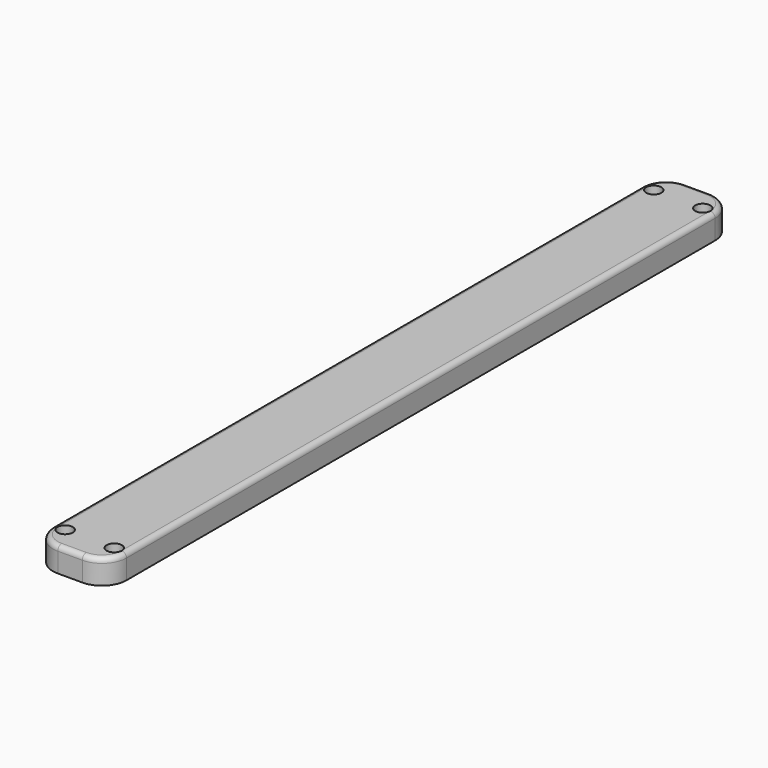
from build123d import *

# Parameters (mm, degrees)
F0_W         = 15
F0_H         = 160
F0_R         = 1.55
F1_DEPTH     = 5
F2_R         = 5
F3_T1_DEPTH  = 150
F3_T3_DEPTH  = 5
F3_T6_ANGLE  = 90
F3_T8_ANGLE  = 90
F3_T10_ANGLE = 90
F3_T12_ANGLE = 90


# Not quite as in the source:
# - a fillet or chamfer that OpenCascade refuses, or shapes differently, is made with other operations: its cross-section is extruded or revolved along the edge and cut away or added


with BuildPart() as f1:
    # F0 (on Top) → F1 (new body)
    with BuildSketch(Plane.XY):
        Rectangle(F0_W, F0_H)
        with Locations((-5, -75)):
            Circle(F0_R, mode=Mode.SUBTRACT)
        with BuildLine():
            ThreePointArc((6.55, -75), (5, -76.55), (3.45, -75))
            ThreePointArc((3.45, -75), (5, -73.45), (6.55, -75))
        make_face(mode=Mode.SUBTRACT)
        with Locations((-5, 75)):
            Circle(F0_R, mode=Mode.SUBTRACT)
        with BuildLine():
            ThreePointArc((6.55, 75), (5, 73.45), (3.45, 75))
            ThreePointArc((3.45, 75), (5, 76.55), (6.55, 75))
        make_face(mode=Mode.SUBTRACT)
    extrude(amount=F1_DEPTH)

    # F2
    f2_edges = [f1.edges().sort_by_distance(p)[0] for p in [
        (7.5, -80, 2.5),
        (-7.5, -80, 2.5),
        (7.5, 80, 2.5),
        (-7.5, 80, 2.5),
    ]]
    fillet(f2_edges, radius=F2_R)

    # F3: fillet of radius 1 on 8 edges, made by hand

    # F3_s2 → F3_t1 (cut)
    with BuildSketch(Plane.XZ.offset(-75)):
        with BuildLine():
            ThreePointArc((6.5, 5), (7.2071067812, 4.7071067812), (7.5, 4))
            Line((7.5, 4), (7.5, 5))
            Line((7.5, 5), (6.5, 5))
        make_face()
        with BuildLine():
            ThreePointArc((-7.5, 4), (-7.2071067812, 4.7071067812), (-6.5, 5))
            Line((-6.5, 5), (-7.5, 5))
            Line((-7.5, 5), (-7.5, 4))
        make_face()
    extrude(amount=F3_T1_DEPTH, mode=Mode.SUBTRACT)

    # F3_s4 → F3_t3 (cut)
    with BuildSketch(Plane.YZ.offset(-2.5)):
        with BuildLine():
            ThreePointArc((79, 5), (79.7071067812, 4.7071067812), (80, 4))
            Line((80, 4), (80, 5))
            Line((80, 5), (79, 5))
        make_face()
        with BuildLine():
            ThreePointArc((-79, 5), (-79.7071067812, 4.7071067812), (-80, 4))
            Line((-80, 4), (-80, 5))
            Line((-80, 5), (-79, 5))
        make_face()
    extrude(amount=F3_T3_DEPTH, mode=Mode.SUBTRACT)

    # F3_s5 → F3_t6 (revolve, cut)
    with BuildSketch(Plane.XZ.offset(-75)):
        with BuildLine():
            ThreePointArc((-7.5, 4), (-7.2071067812, 4.7071067812), (-6.5, 5))
            Line((-6.5, 5), (-7.5, 5))
            Line((-7.5, 5), (-7.5, 4))
        make_face()
    revolve(axis=Axis((-2.5, 75, 5), (0, 0, -1)), revolution_arc=F3_T6_ANGLE, mode=Mode.SUBTRACT)

    # F3_s7 → F3_t8 (revolve, cut)
    with BuildSketch(Plane.XZ.offset(75)):
        with BuildLine():
            ThreePointArc((-7.5, 4), (-7.2071067812, 4.7071067812), (-6.5, 5))
            Line((-6.5, 5), (-7.5, 5))
            Line((-7.5, 5), (-7.5, 4))
        make_face()
    revolve(axis=Axis((-2.5, -75, 5), (0, 0, 1)), revolution_arc=F3_T8_ANGLE, mode=Mode.SUBTRACT)

    # F3_s9 → F3_t10 (revolve, cut)
    with BuildSketch(Plane.XZ.offset(-75)):
        with BuildLine():
            ThreePointArc((6.5, 5), (7.2071067812, 4.7071067812), (7.5, 4))
            Line((7.5, 4), (7.5, 5))
            Line((7.5, 5), (6.5, 5))
        make_face()
    revolve(axis=Axis((2.5, 75, 5), (0, 0, 1)), revolution_arc=F3_T10_ANGLE, mode=Mode.SUBTRACT)

    # F3_s11 → F3_t12 (revolve, cut)
    with BuildSketch(Plane.XZ.offset(75)):
        with BuildLine():
            ThreePointArc((6.5, 5), (7.2071067812, 4.7071067812), (7.5, 4))
            Line((7.5, 4), (7.5, 5))
            Line((7.5, 5), (6.5, 5))
        make_face()
    revolve(axis=Axis((2.5, -75, 5), (0, 0, -1)), revolution_arc=F3_T12_ANGLE, mode=Mode.SUBTRACT)


solid = f1.part
